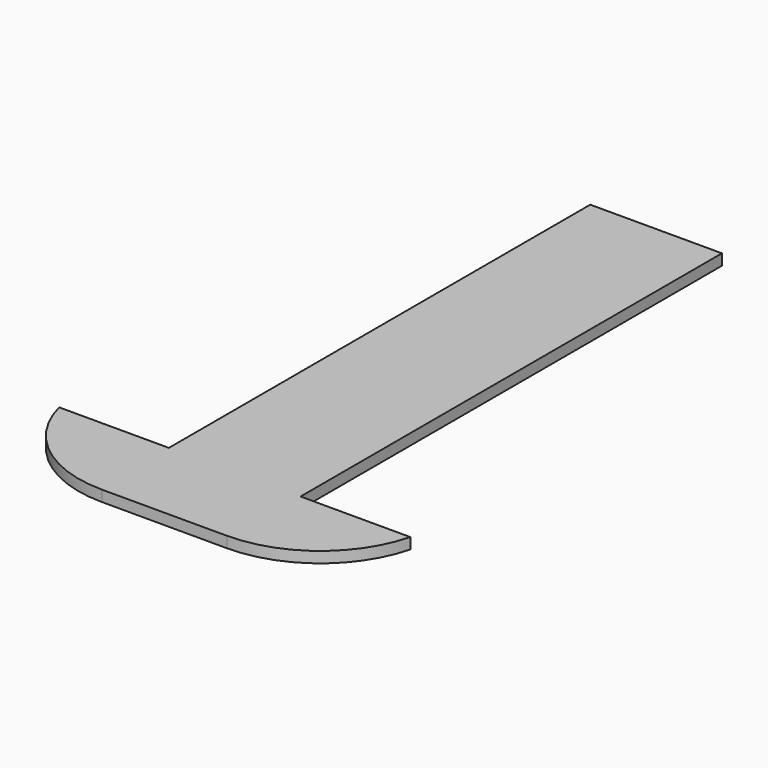
from build123d import *

# Parameters (mm, degrees)
F1_DEPTH    = 3.175
F2_T1_DEPTH = 166.5877767412


# Not quite as in the source:
# - a fillet or chamfer that OpenCascade refuses, or shapes differently, is made with other operations: its cross-section is extruded or revolved along the edge and cut away or added


with BuildPart() as f1:
    # F0 (on Top) → F1 (new body)
    with BuildSketch(Plane.XY):
        Polygon((19.05, -76.2), (19.05, 76.2), (-19.05, 76.2), (-19.05, -76.2), (-50.8, -76.2), (-50.8, -101.6), (50.8, -101.6), (50.8, -76.2), align=None)
    extrude(amount=F1_DEPTH)

    # F2: fillet of radius 33.7265634664 on 2 edges, made by hand

    # F2_s2 → F2_t1 (cut)
    with BuildSketch(Plane.XY.offset(-81.7063883706)):
        with BuildLine():
            ThreePointArc((-50.8, -76.2), (-38.8135156804, -94.5033769622), (-18.1174446518, -101.6))
            Line((-18.1174446518, -101.6), (-50.8, -101.6))
            Line((-50.8, -101.6), (-50.8, -76.2))
        make_face()
        with BuildLine():
            ThreePointArc((18.1174446518, -101.6), (38.8135156804, -94.5033769622), (50.8, -76.2))
            Line((50.8, -76.2), (50.8, -101.6))
            Line((50.8, -101.6), (18.1174446518, -101.6))
        make_face()
    extrude(amount=F2_T1_DEPTH, mode=Mode.SUBTRACT)


solid = f1.part
